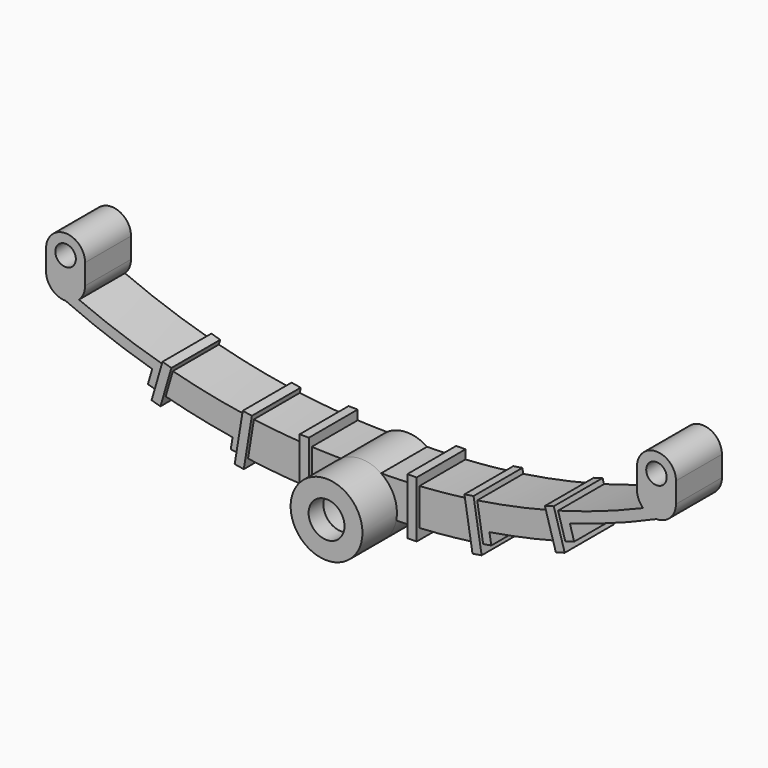
from build123d import *

# Parameters (mm, degrees)
F0_R     = 1.75
F0_R_2   = 1
F1_DEPTH = 5.6
F3_W     = 0.9
F3_H     = 5.5
F4_DEPTH = 5.95
F5_R     = 3.5
F5_R_2   = 1.75
F6_DEPTH = 4.2
F7_R     = 2.5
F8_DEPTH = 8


with BuildPart() as f1:
    # F0 (on Front) → F1 (new body)
    with BuildSketch(Plane.XZ):
        with BuildLine():
            Line((-26.9, -2), (-26.9, 0))
            ThreePointArc((-26.9, 0), (-28.8, 1.9), (-30.7, 0))
            Line((-30.7, 0), (-30.7, -2))
            ThreePointArc((-30.7, -2), (-30.1435028843, -3.3435028843), (-28.8, -3.9))
            ThreePointArc((-28.8, -3.9), (-24.6294135718, -5.596855554), (-20.3538194655, -7.0083813116))
            Line((-20.3538194655, -7.0083813116), (-20.7757003916, -8.4478313747))
            ThreePointArc((-20.7757003916, -8.4478313747), (-16.6769659984, -9.5120684601), (-12.5200691265, -10.3198014574))
            Line((-12.5200691265, -10.3198014574), (-12.696252722, -11.4056003986))
            ThreePointArc((-12.696252722, -11.4056003986), (-8.0798243817, -11.9962992417), (-3.4341530829, -12.2757163632))
            ThreePointArc((-3.4341530829, -12.2757163632), (0, -15.1), (3.4341530829, -12.2757163632))
            ThreePointArc((3.4341530829, -12.2757163632), (3.235336932, -10.2648614543), (1.9581459203, -8.699023517))
            ThreePointArc((1.9581459203, -8.699023517), (0, -8.1), (-1.9581459203, -8.699023517))
            ThreePointArc((-1.9581459203, -8.699023517), (-14.9928565077, -7.3200147056), (-27.4941674529, -3.3801454123))
            ThreePointArc((-27.4941674529, -3.3801454123), (-27.0548521783, -2.7513049183), (-26.9, -2))
        make_face()
        with Locations((0, -11.6)):
            Circle(F0_R, mode=Mode.SUBTRACT)
        with Locations((-28.8, 0)):
            Circle(F0_R_2, mode=Mode.SUBTRACT)
        with BuildLine():
            ThreePointArc((27.4941674529, -3.3801454123), (14.9928565077, -7.3200147056), (1.9581459203, -8.699023517))
            ThreePointArc((1.9581459203, -8.699023517), (3.235336932, -10.2648614543), (3.4341530829, -12.2757163632))
            ThreePointArc((3.4341530829, -12.2757163632), (8.0798243817, -11.9962992417), (12.696252722, -11.4056003986))
            Line((12.696252722, -11.4056003986), (12.5200691265, -10.3198014574))
            ThreePointArc((12.5200691265, -10.3198014574), (16.6769659984, -9.5120684601), (20.7757003916, -8.4478313747))
            Line((20.7757003916, -8.4478313747), (20.3538194655, -7.0083813116))
            ThreePointArc((20.3538194655, -7.0083813116), (24.6294135718, -5.596855554), (28.8, -3.9))
            ThreePointArc((28.8, -3.9), (30.1435028843, -3.3435028843), (30.7, -2))
            Line((30.7, -2), (30.7, 0))
            ThreePointArc((30.7, 0), (28.8, 1.9), (26.9, 0))
            Line((26.9, 0), (26.9, -2))
            ThreePointArc((26.9, -2), (27.0548521783, -2.7513049183), (27.4941674529, -3.3801454123))
        make_face()
        with Locations((28.8, 0)):
            Circle(F0_R_2, mode=Mode.SUBTRACT)
    extrude(amount=F1_DEPTH)

    # F3 (on offset) → F4 (join, through all)
    with BuildSketch(Plane.XZ.offset(5.95)):
        Polygon((-18.2045984637, -6.0751883598), (-19.0682685015, -5.8220598041), (-20.1370335143, -9.4686666307), (-19.2733634764, -9.7217951863), align=None)
        Polygon((-10.3615155022, -7.6308153564), (-11.2498964541, -7.4866651419), (-12.0347142888, -12.3234058798), (-11.146333337, -12.4675560944), align=None)
        with Locations((-5.25, -10.45)):
            Rectangle(F3_W, F3_H)
        with Locations((5.25, -10.45)):
            Rectangle(F3_W, F3_H)
        Polygon((11.146333337, -12.4675560944), (12.0347142888, -12.3234058798), (11.2498964541, -7.4866651419), (10.3615155022, -7.6308153564), align=None)
        Polygon((20.1370335143, -9.4686666307), (19.0682685015, -5.8220598041), (18.2045984637, -6.0751883598), (19.2733634764, -9.7217951863), align=None)
    extrude(amount=-F4_DEPTH)

    # F5 (on face) → F6 (join)
    with BuildSketch(Plane.XZ.offset(5.6)):
        with Locations((0, -11.6)):
            Circle(F5_R)
        with Locations((0, -11.6)):
            Circle(F5_R_2, mode=Mode.SUBTRACT)
    extrude(amount=F6_DEPTH)

    # F7 (on face) → F8 (cut)
    with BuildSketch(Plane(origin=(0, 0, 0), x_dir=(-1, 0, 0), z_dir=(0, 1, 0))):
        with Locations((0, -11.6)):
            Circle(F7_R)
    extrude(amount=-F8_DEPTH, mode=Mode.SUBTRACT)


solid = f1.part
